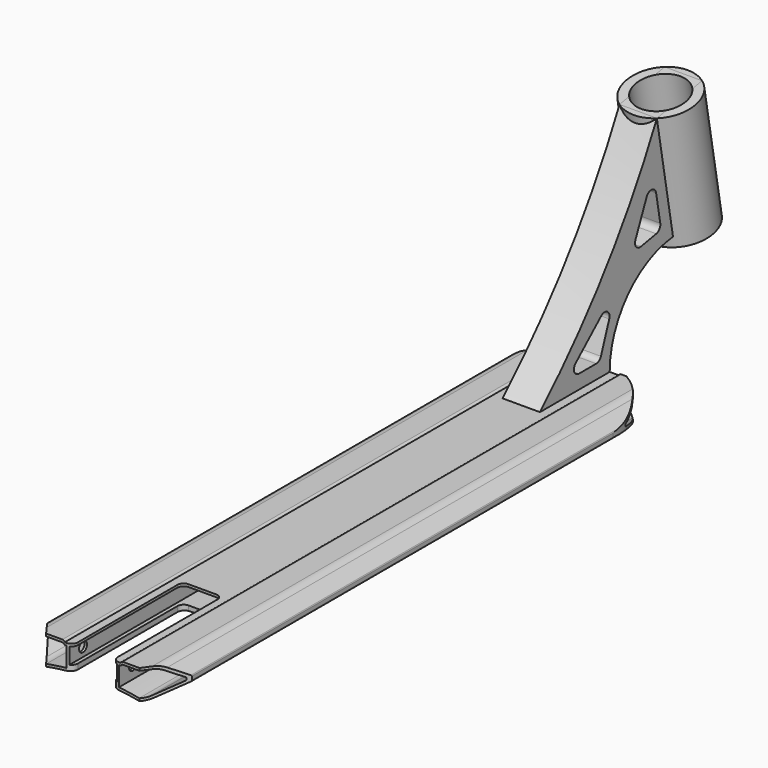
from build123d import *

# Parameters (mm, degrees)
F1_DEPTH       = 250
F2_W           = 38
F2_H           = 13
F3_DEPTH       = 250
F4_T1_DEPTH    = 509.3674969976
F5_R           = 9
F6_R           = 1
F8_DEPTH       = 500.001
F10_DEPTH      = 13.5193051812
F10_DEPTH_BACK = 10.001
F12_DEPTH      = 13.519305294
F12_DEPTH_BACK = 10.0010001
F13_F1_R       = 4.9999
F13_F2_R       = 4.9999
F13_F3_R       = 5
F13_F4_R       = 5
F13_F5_R       = 5
F13_F6_R       = 5
F15_DEPTH      = 15
F16_R          = 27.5
F17_DEPTH      = 100
F19_D          = 40
F21_D          = 8
F21_DEPTH      = 78.5010001
F23_DEPTH      = 72.5010001
F24_R          = 5


# Not quite as in the source:
# - a fillet or chamfer that OpenCascade refuses, or shapes differently, is made with other operations: its cross-section is extruded or revolved along the edge and cut away or added
# - a fillet or chamfer is up to 0.001 mm smaller than in the source, because OpenCascade refuses the exact size


with BuildPart() as f1:
    # F0 (on Front) → F1 (new body, symmetric)
    with BuildSketch(Plane.XZ):
        with BuildLine():
            Line((22.5, 8.7), (0, 8.7))
            Line((0, 8.7), (-22.5, 8.7))
            Line((-22.5, 8.7), (-22.5, 10))
            Line((-22.5, 10), (-45.5824640741, 10))
            Line((-45.5824640741, 10), (-57.5, 0))
            Line((-57.5, 0), (-57.5, -4))
            Line((-57.5, -4), (-40.1794919243, -14))
            ThreePointArc((-40.1794919243, -14), (0, -9.9224551416), (40.1794919243, -14))
            Line((40.1794919243, -14), (57.5, -4))
            Line((57.5, -4), (57.5, 0))
            Line((57.5, 0), (45.5824640741, 10))
            Line((45.5824640741, 10), (22.5, 10))
            Line((22.5, 10), (22.5, 8.7))
        make_face()
    extrude(amount=F1_DEPTH, both=True)

    # F2 (on Front) → F3 (cut, symmetric)
    with BuildSketch(Plane.XZ):
        with Locations((0, 0.2)):
            Rectangle(F2_W, F2_H)
    extrude(amount=F3_DEPTH, both=True, mode=Mode.SUBTRACT)

    # F4: fillet of radius 2 on 2 edges, made by hand

    # F4_s2 → F4_t1 (cut)
    with BuildSketch(Plane.XZ.offset(-254.6837484988)):
        with BuildLine():
            ThreePointArc((-24.3734993995, 10), (-23.2333239744, 9.6431676725), (-22.5, 8.7))
            Line((-22.5, 8.7), (-22.5, 10))
            Line((-22.5, 10), (-24.3734993995, 10))
        make_face()
        with BuildLine():
            ThreePointArc((24.3734993995, 10), (23.2333239744, 9.6431676725), (22.5, 8.7))
            Line((22.5, 8.7), (22.5, 10))
            Line((22.5, 10), (24.3734993995, 10))
        make_face()
    extrude(amount=F4_T1_DEPTH, mode=Mode.SUBTRACT)

    # F5
    f5_edges = [f1.edges().sort_by_distance(p)[0] for p in [
        (-45.582464, 0, 10),
        (45.582464, 0, 10),
        (-40.179492, 0, -14),
        (40.179492, 0, -14),
    ]]
    fillet(f5_edges, radius=F5_R)

    # F6
    f6_edges = [f1.edges().sort_by_distance(p)[0] for p in [
        (-57.5, 0, 0),
        (-57.5, 0, -4),
        (57.5, 0, 0),
        (57.5, 0, -4),
    ]]
    fillet(f6_edges, radius=F6_R)

    # F7 (on face) → F8 (cut, through all)
    with BuildSketch(Plane.XZ.offset(250)):
        with BuildLine():
            ThreePointArc((-22.5, 6.7), (-23.2333239744, 7.6431676725), (-24.3734993995, 8))
            Line((-24.3734993995, 8), (-42.3067319657, 8))
            ThreePointArc((-42.3067319657, 8), (-44.7008729689, 7.5778483455), (-46.8062452335, 6.3623111018))
            Line((-46.8062452335, 6.3623111018), (-55.1427876097, -0.6328785313))
            ThreePointArc((-55.1427876097, -0.6328785313), (-55.406307787, -0.9763047127), (-55.5, -1.3989229745))
            Line((-55.5, -1.3989229745), (-55.5, -2.2679491924))
            ThreePointArc((-55.5, -2.2679491924), (-55.3660254038, -2.7679491924), (-55, -3.1339745962))
            Line((-55, -3.1339745962), (-42.1022690923, -10.5804830077))
            ThreePointArc((-42.1022690923, -10.5804830077), (-39.7790673433, -11.4186780608), (-37.3093701274, -11.3978700124))
            ThreePointArc((-37.3093701274, -11.3978700124), (-29.1789785809, -10.0410222645), (-21, -9.0170047426))
            Line((-21, -9.0170047426), (-21, 6.7))
            Line((-21, 6.7), (-22.5, 6.7))
        make_face()
        with BuildLine():
            ThreePointArc((55, -3.1339745962), (55.3660254038, -2.7679491924), (55.5, -2.2679491924))
            Line((55.5, -2.2679491924), (55.5, -1.3989229745))
            ThreePointArc((55.5, -1.3989229745), (55.406307787, -0.9763047127), (55.1427876097, -0.6328785313))
            Line((55.1427876097, -0.6328785313), (46.8062452335, 6.3623111018))
            ThreePointArc((46.8062452335, 6.3623111018), (44.7008729689, 7.5778483455), (42.3067319657, 8))
            Line((42.3067319657, 8), (24.3734993995, 8))
            ThreePointArc((24.3734993995, 8), (23.2333239744, 7.6431676725), (22.5, 6.7))
            Line((22.5, 6.7), (21, 6.7))
            Line((21, 6.7), (21, -9.0170047426))
            ThreePointArc((21, -9.0170047426), (29.1789785809, -10.0410222645), (37.3093701274, -11.3978700124))
            ThreePointArc((37.3093701274, -11.3978700124), (39.7790673433, -11.4186780608), (42.1022690923, -10.5804830077))
            Line((42.1022690923, -10.5804830077), (55, -3.1339745962))
        make_face()
    extrude(amount=-F8_DEPTH, mode=Mode.SUBTRACT)

    # F9 (on Top) → F10 (cut, two sides)
    with BuildSketch(Plane.XY) as f10_sk:
        with BuildLine():
            ThreePointArc((-57.5, 200), (0, 257.5), (57.5, 200))
            Line((57.5, 200), (57.5, 280))
            Line((57.5, 280), (-57.5, 280))
            Line((-57.5, 280), (-57.5, 200))
        make_face()
    extrude(amount=-F10_DEPTH, mode=Mode.SUBTRACT)
    extrude(f10_sk.sketch, amount=F10_DEPTH_BACK, mode=Mode.SUBTRACT)

    # F11 (on Top) → F12 (cut, two sides)
    with BuildSketch(Plane.XY) as f12_sk:
        Polygon((16, -250), (16, -140), (-16, -140), (-16, -250), (-37.4852138238, -250), (-68, -208), (-68, -338), (68, -338), (68, -208), (37.4852138238, -250), align=None)
    extrude(amount=-F12_DEPTH, mode=Mode.SUBTRACT)
    extrude(f12_sk.sketch, amount=F12_DEPTH_BACK, mode=Mode.SUBTRACT)

    # F13: fillet of radius 5 on 8 edges, made by hand

    # F13_f1 (radius 5 in the source; OpenCascade refuses exactly that, so slightly less here)
    f13_f1_edges = [f1.edges().sort_by_distance(p)[0] for p in [
        (16, -250, -8.4317412158),
    ]]
    fillet(f13_f1_edges, radius=F13_F1_R)

    # F13_f2 (radius 5 in the source; OpenCascade refuses exactly that, so slightly less here)
    f13_f2_edges = [f1.edges().sort_by_distance(p)[0] for p in [
        (-16, -250, 7.7),
    ]]
    fillet(f13_f2_edges, radius=F13_F2_R)

    # F13_f3
    f13_f3_edges = [f1.edges().sort_by_distance(p)[0] for p in [
        (-16, -140, -8.4317412158),
    ]]
    fillet(f13_f3_edges, radius=F13_F3_R)

    # F13_f4
    f13_f4_edges = [f1.edges().sort_by_distance(p)[0] for p in [
        (16, -140, -8.4317412158),
    ]]
    fillet(f13_f4_edges, radius=F13_F4_R)

    # F13_f5
    f13_f5_edges = [f1.edges().sort_by_distance(p)[0] for p in [
        (16, -140, 7.7),
    ]]
    fillet(f13_f5_edges, radius=F13_F5_R)

    # F13_f6
    f13_f6_edges = [f1.edges().sort_by_distance(p)[0] for p in [
        (-16, -140, 7.7),
    ]]
    fillet(f13_f6_edges, radius=F13_F6_R)

    # F14 (on Right) → F15 (join, symmetric)
    with BuildSketch(Plane.YZ):
        with BuildLine():
            ThreePointArc((297.3819995028, 168.7), (245.9666940414, 83.362277853), (180, 8.7))
            Line((180, 8.7), (250, 8.7))
            ThreePointArc((250, 8.7), (268.2890377472, 55.8802483656), (313.5993194522, 78.4067463039))
            Line((313.5993194522, 78.4067463039), (315.0598515595, 70.2749343578))
            Line((315.0598515595, 70.2749343578), (360.3353817549, 78.4067463039))
            Line((360.3353817549, 78.4067463039), (342.6575296982, 176.8318119461))
            Line((342.6575296982, 176.8318119461), (297.3819995028, 168.7))
        make_face()
    extrude(amount=F15_DEPTH, both=True)

    # F16 (on face) → F17 (join, through all)
    with BuildSketch(Plane(origin=(0, -20.0594716521, 111.6852210195), x_dir=(1, 0, 0), z_dir=(0, -0.1767785206, 0.9842506564))):
        with Locations((0, 345.5209646382)):
            Circle(F16_R)
    extrude(amount=-F17_DEPTH)

    # F19 (through all)
    with Locations(Plane(origin=(0, -20.0594716521, 111.6852210195), x_dir=(1, 0, 0), z_dir=(0, -0.1767785206, 0.9842506564))):
        with Locations((0, 345.5209646382)):
            Hole(F19_D / 2)

    # F21 (through all, one way)
    with BuildSketch(Plane.YZ.offset(21)):
        with Locations((-236, 0.9829952574)):
            Circle(F21_D / 2)
    extrude(amount=-F21_DEPTH, mode=Mode.SUBTRACT)

    # F22 (on face) → F23 (cut, through all)
    with BuildSketch(Plane.YZ.offset(15)):
        Polygon((301.6336829716, 88.18352468), (293.6786495461, 132.474804219), (272.106163279, 82.880169063), align=None)
        Polygon((206, 20), (240, 20), (256.378660542, 65), align=None)
    extrude(amount=-F23_DEPTH, mode=Mode.SUBTRACT)

    # F24
    f24_edges = [f1.edges().sort_by_distance(p)[0] for p in [
        (0, 293.67865, 132.474804),
        (0, 301.633683, 88.183525),
        (0, 272.106163, 82.880169),
        (0, 240, 20),
        (0, 256.378661, 65),
        (0, 206, 20),
    ]]
    fillet(f24_edges, radius=F24_R)


solid = f1.part
